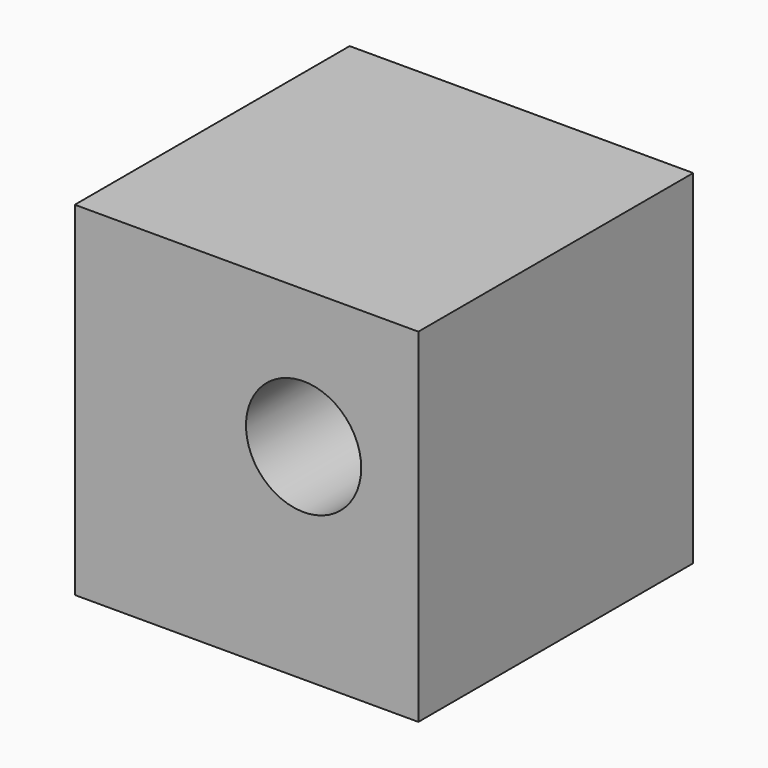
from build123d import *

# Parameters (mm, degrees)
F0_W     = 25.4
F0_H     = 25.4
F2_DEPTH = 25.4
F5_R     = 4.2589034539
F6_DEPTH = 38.862


# Not quite as in the source:
# - a feature of the source that left no trace in its solid (it failed there, or was rolled back) is left out


with BuildPart() as f2:
    # F0 (on Front) → F2 (new body)
    with BuildSketch(Plane.XZ):
        with Locations((-12.7, 12.7)):
            Rectangle(F0_W, F0_H)
    extrude(amount=F2_DEPTH)

    # F5 (on Front) → F6 (cut)
    with BuildSketch(Plane.XZ):
        with Locations((-8.4840552881, 15.1530262083)):
            Circle(F5_R)
    extrude(amount=F6_DEPTH, mode=Mode.SUBTRACT)


solid = f2.part
